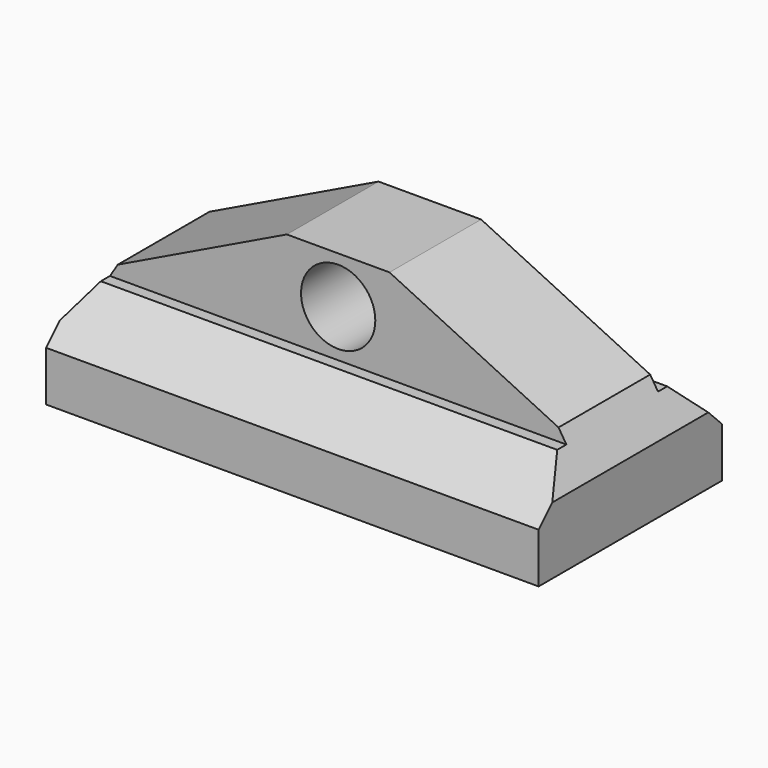
from build123d import *

# Parameters (mm, degrees)
F0_R        = 4.1158301742
F1_DEPTH    = 6.35
F0_W        = 54.6039827168
F0_H        = 10.6174414977
F2_DEPTH    = 12.7
F3_T1_DEPTH = 80.7322818745
F3_T3_DEPTH = 29.5163540068
F3_T5_DEPTH = 29.5163538598


# Not quite as in the source:
# - a fillet or chamfer that OpenCascade refuses, or shapes differently, is made with other operations: its cross-section is extruded or revolved along the edge and cut away or added


with BuildPart() as f1:
    # F0 (on Front) → F1 (new body, symmetric)
    with BuildSketch(Plane.XZ):
        Polygon((-5.6879152544, 15.7365649939), (-27.3019913584, 5.3087207489), (27.3019913584, 5.3087207489), (5.68791572, 15.7365649939), (0, 15.7365649939), align=None)
        with Locations((0, 10.5226428714)):
            Circle(F0_R, mode=Mode.SUBTRACT)
    extrude(amount=F1_DEPTH, both=True)

    # F0 (on Front) → F2 (join, symmetric)
    with BuildSketch(Plane.XZ):
        Rectangle(F0_W, F0_H)
    extrude(amount=F2_DEPTH, both=True)

    # F3: chamfer of 5.08 on 4 edges, made by hand

    # F3_s2 → F3_t1 (cut)
    with BuildSketch(Plane.YZ.offset(-40.3661409373)):
        Polygon((-7.62, 5.3087207489), (-12.7, 0.2287207489), (-12.7, 5.3087207489), align=None)
        Polygon((7.62, 5.3087207489), (12.7, 0.2287207489), (12.7, 5.3087207489), align=None)
    extrude(amount=F3_T1_DEPTH, mode=Mode.SUBTRACT)

    # F3_s4 → F3_t3 (cut)
    with BuildSketch(Plane.XZ.offset(-14.7581770034)):
        Polygon((-27.3019913584, 2.1192789571), (-24.4293942586, 6.6946229263), (-27.3019913584, 5.3087207489), align=None)
    extrude(amount=F3_T3_DEPTH, mode=Mode.SUBTRACT)

    # F3_s6 → F3_t5 (cut)
    with BuildSketch(Plane.XZ.offset(-14.7581769299)):
        Polygon((27.3019913584, 2.119278987), (24.4293942972, 6.6946229375), (27.3019913584, 5.3087207489), align=None)
    extrude(amount=F3_T5_DEPTH, mode=Mode.SUBTRACT)


solid = f1.part
